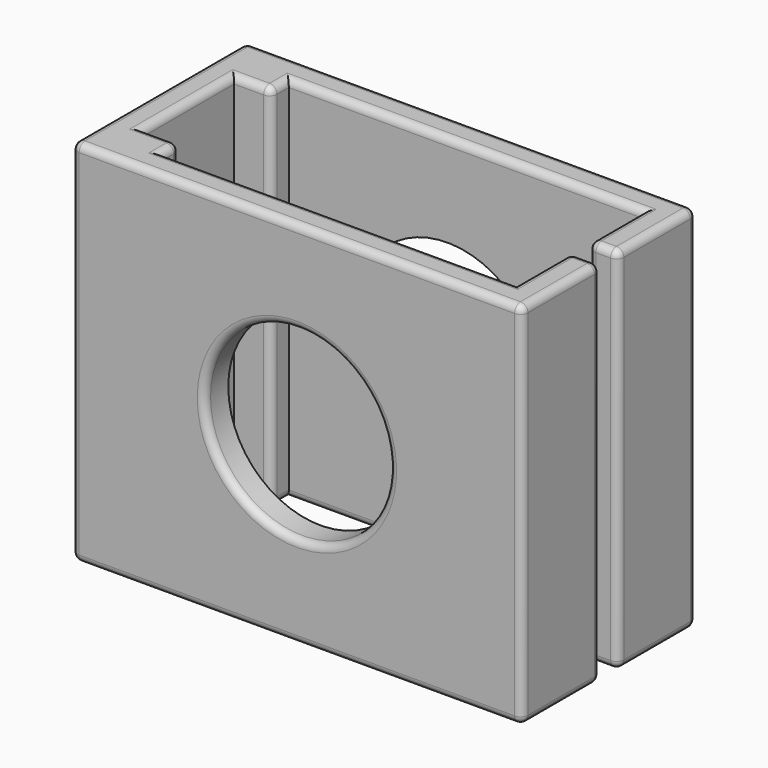
from build123d import *

# Parameters (mm, degrees)
F1_DEPTH = 50
F2_R     = 12.5
F3_DEPTH = 29.501
F6_F1_R  = 1
F6_F2_R  = 1
F6_F3_R  = 1
F6_F4_R  = 1
F6_F5_R  = 1
F6_F6_R  = 1
F6_F7_R  = 1
F6_F8_R  = 1
F6_F9_R  = 1
F6_F10_R = 1
F6_F11_R = 1
F6_F12_R = 1
F6_F13_R = 1
F6_F14_R = 1
F6_F15_R = 1
F6_F16_R = 1
F6_F17_R = 1
F6_F18_R = 1
F6_F19_R = 1
F6_F20_R = 1
F6_F21_R = 1
F6_F22_R = 1
F6_F23_R = 1
F6_F24_R = 1
F6_F25_R = 1


# Not quite as in the source:
# - a feature of the source that left no trace in its solid (it failed there, or was rolled back) is left out


with BuildPart() as f1:
    # F0 (on Top) → F1 (new body)
    with BuildSketch(Plane.XY):
        Polygon((0, 0), (61, 0), (61, 13.25), (57, 13.25), (57, 4), (9, 4), (9, 7), (4, 7), (4, 22.5), (9, 22.5), (9, 25.5), (57, 25.5), (57, 16.25), (61, 16.25), (61, 29.5), (0, 29.5), align=None)
    extrude(amount=F1_DEPTH)

    # F2 (on face) → F3 (cut, through all)
    with BuildSketch(Plane(origin=(0, 29.5, 0), x_dir=(-1, 0, 0), z_dir=(0, 1, 0))):
        with Locations((-30.5, 25)):
            Circle(F2_R)
    extrude(amount=-F3_DEPTH, mode=Mode.SUBTRACT)

    # F6: fillet of radius 1 on 36 edges, made by hand

    # F6_f1
    f6_f1_edges = [f1.edges().sort_by_distance(p)[0] for p in [
        (43, 0, 25),
    ]]
    fillet(f6_f1_edges, radius=F6_F1_R)

    # F6_f2
    f6_f2_edges = [f1.edges().sort_by_distance(p)[0] for p in [
        (43, 29.5, 25),
    ]]
    fillet(f6_f2_edges, radius=F6_F2_R)

    # F6_f3
    f6_f3_edges = [f1.edges().sort_by_distance(p)[0] for p in [
        (30.5, 0, 0),
    ]]
    fillet(f6_f3_edges, radius=F6_F3_R)

    # F6_f4
    f6_f4_edges = [f1.edges().sort_by_distance(p)[0] for p in [
        (30.5, 0, 50),
    ]]
    fillet(f6_f4_edges, radius=F6_F4_R)

    # F6_f5
    f6_f5_edges = [f1.edges().sort_by_distance(p)[0] for p in [
        (30.5, 29.5, 0),
    ]]
    fillet(f6_f5_edges, radius=F6_F5_R)

    # F6_f6
    f6_f6_edges = [f1.edges().sort_by_distance(p)[0] for p in [
        (30.5, 29.5, 50),
    ]]
    fillet(f6_f6_edges, radius=F6_F6_R)

    # F6_f7
    f6_f7_edges = [f1.edges().sort_by_distance(p)[0] for p in [
        (0, 0, 25),
    ]]
    fillet(f6_f7_edges, radius=F6_F7_R)

    # F6_f8
    f6_f8_edges = [f1.edges().sort_by_distance(p)[0] for p in [
        (61, 0, 25),
    ]]
    fillet(f6_f8_edges, radius=F6_F8_R)

    # F6_f9
    f6_f9_edges = [f1.edges().sort_by_distance(p)[0] for p in [
        (61, 13.25, 25),
    ]]
    fillet(f6_f9_edges, radius=F6_F9_R)

    # F6_f10
    f6_f10_edges = [f1.edges().sort_by_distance(p)[0] for p in [
        (61, 29.5, 25),
    ]]
    fillet(f6_f10_edges, radius=F6_F10_R)

    # F6_f11
    f6_f11_edges = [f1.edges().sort_by_distance(p)[0] for p in [
        (57, 13.25, 25),
    ]]
    fillet(f6_f11_edges, radius=F6_F11_R)

    # F6_f12
    f6_f12_edges = [f1.edges().sort_by_distance(p)[0] for p in [
        (9, 7, 25),
    ]]
    fillet(f6_f12_edges, radius=F6_F12_R)

    # F6_f13
    f6_f13_edges = [f1.edges().sort_by_distance(p)[0] for p in [
        (9, 22.5, 25),
    ]]
    fillet(f6_f13_edges, radius=F6_F13_R)

    # F6_f14
    f6_f14_edges = [f1.edges().sort_by_distance(p)[0] for p in [
        (57, 16.25, 25),
    ]]
    fillet(f6_f14_edges, radius=F6_F14_R)

    # F6_f15
    f6_f15_edges = [f1.edges().sort_by_distance(p)[0] for p in [
        (61, 16.25, 25),
    ]]
    fillet(f6_f15_edges, radius=F6_F15_R)

    # F6_f16
    f6_f16_edges = [f1.edges().sort_by_distance(p)[0] for p in [
        (33, 4, 0),
    ]]
    fillet(f6_f16_edges, radius=F6_F16_R)

    # F6_f17
    f6_f17_edges = [f1.edges().sort_by_distance(p)[0] for p in [
        (33, 25.5, 0),
    ]]
    fillet(f6_f17_edges, radius=F6_F17_R)

    # F6_f18
    f6_f18_edges = [f1.edges().sort_by_distance(p)[0] for p in [
        (33, 4, 50),
    ]]
    fillet(f6_f18_edges, radius=F6_F18_R)

    # F6_f19
    f6_f19_edges = [f1.edges().sort_by_distance(p)[0] for p in [
        (33, 25.5, 50),
    ]]
    fillet(f6_f19_edges, radius=F6_F19_R)

    # F6_f20
    f6_f20_edges = [f1.edges().sort_by_distance(p)[0] for p in [
        (4, 14.75, 0),
    ]]
    fillet(f6_f20_edges, radius=F6_F20_R)

    # F6_f21
    f6_f21_edges = [f1.edges().sort_by_distance(p)[0] for p in [
        (4, 14.75, 50),
    ]]
    fillet(f6_f21_edges, radius=F6_F21_R)

    # F6_f22
    f6_f22_edges = [f1.edges().sort_by_distance(p)[0] for p in [
        (6, 7, 0),
    ]]
    fillet(f6_f22_edges, radius=F6_F22_R)

    # F6_f23
    f6_f23_edges = [f1.edges().sort_by_distance(p)[0] for p in [
        (6, 22.5, 0),
    ]]
    fillet(f6_f23_edges, radius=F6_F23_R)

    # F6_f24
    f6_f24_edges = [f1.edges().sort_by_distance(p)[0] for p in [
        (6, 7, 50),
    ]]
    fillet(f6_f24_edges, radius=F6_F24_R)

    # F6_f25
    f6_f25_edges = [f1.edges().sort_by_distance(p)[0] for p in [
        (6, 22.5, 50),
    ]]
    fillet(f6_f25_edges, radius=F6_F25_R)


solid = f1.part
